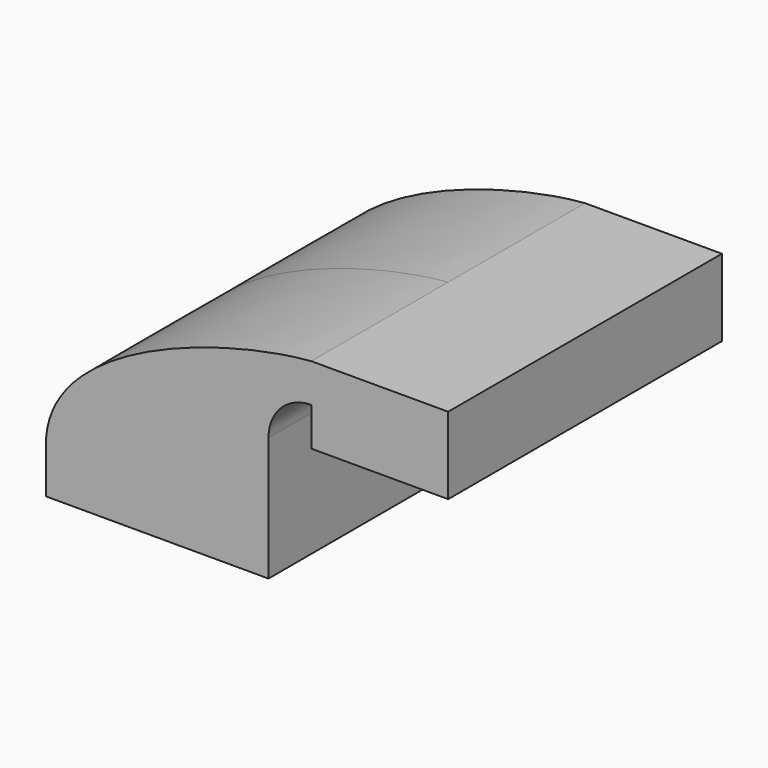
from build123d import *

# Parameters (mm, degrees)
F0_W     = 25.4
F0_H     = 13.97
F1_DEPTH = 63.5


with BuildPart() as f1:
    # F0 (on Front) → F1 (new body, symmetric)
    with BuildSketch(Plane.XZ):
        with BuildLine():
            add(Edge.make_bspline(
                [(-41.275, 9.525), (-38.7320481241, 45.0227931142), (26.9261933863, 64.3182843924), (57.15, 66.675)],
                knots=[0, 0, 0, 0, 113.8138968887, 113.8138968887, 113.8138968887, 113.8138968887], degree=3))
            Line((-41.275, 9.525), (27.305, 9.525))
            Line((27.305, 9.525), (27.305, 36.5125))
            ThreePointArc((27.305, 36.5125), (36.0463981155, 57.6161018845), (57.15, 66.3575))
            Line((57.15, 66.3575), (57.15, 66.675))
        make_face()
        Polygon((27.305, 9.525), (-41.275, 9.525), (-41.275, -9.525), (41.275, -9.525), (41.275, 9.525), align=None)
        with BuildLine():
            Line((27.305, 36.5125), (27.305, 9.525))
            Line((27.305, 9.525), (41.275, 9.525))
            Line((41.275, 9.525), (41.275, 36.5125))
            ThreePointArc((41.275, 36.5125), (45.9246798487, 47.7378201513), (57.15, 52.3875))
            Line((57.15, 52.3875), (57.15, 66.3575))
            ThreePointArc((57.15, 66.3575), (36.0463981155, 57.6161018845), (27.305, 36.5125))
        make_face()
        Polygon((107.95, 66.675), (57.15, 66.675), (57.15, 66.3575), (82.55, 66.3575), (82.55, 52.3875), (57.15, 52.3875), (57.15, 38.1), (107.95, 38.1), align=None)
        with Locations((69.85, 59.3725)):
            Rectangle(F0_W, F0_H)
    extrude(amount=F1_DEPTH, both=True)


solid = f1.part
